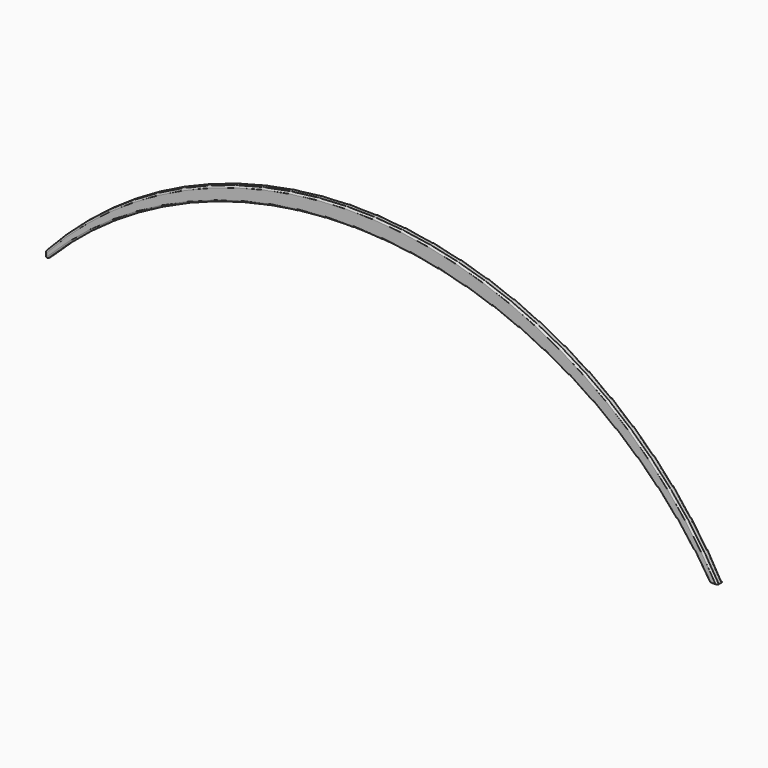
from build123d import *

# Parameters (mm, degrees)
F1_DEPTH = 2
F3_R     = 0.5


# Not quite as in the source:
# - a feature of the source that left no trace in its solid (it failed there, or was rolled back) is left out


with BuildPart() as f1:
    # F0 (on Front) → F1 (new body)
    with BuildSketch(Plane.XZ):
        with BuildLine():
            ThreePointArc((-200, 20), (-95.7942395393, 58.005682078), (-1.25, 0))
            Line((-1.25, 0), (1.25, 0))
            ThreePointArc((1.25, 0), (-93.630783891, 62.6288218635), (-200, 22.5))
            Line((-200, 22.5), (-200, 20))
        make_face()
    extrude(amount=F1_DEPTH)

    # F3
    f3_edges = [f1.edges().sort_by_distance(p)[0] for p in [
        (-200, -1, 22.5),
        (-200, -1, 20),
        (-200, 0, 21.25),
        (-200, -2, 21.25),
        (-93.630784, 0, 62.628822),
        (-93.630784, -2, 62.628822),
        (-95.79424, 0, 58.005682),
        (-95.79424, -2, 58.005682),
    ]]
    fillet(f3_edges, radius=F3_R)


solid = f1.part
